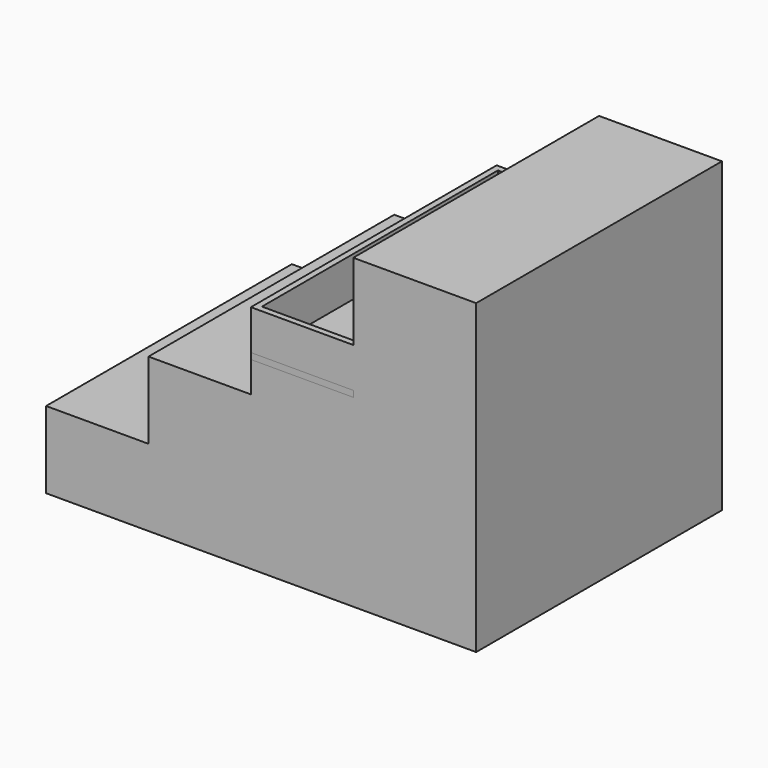
from build123d import *

# Parameters (mm, degrees)
F1_DEPTH = 60
F2_W     = 17.6
F2_H     = 57.6
F3_DEPTH = 25
F4_DEPTH = 16
F5_W     = 20
F5_H     = 60
F5_W_2   = 17.6
F5_H_2   = 57.6
F6_DEPTH = 1.2


with BuildPart() as f1:
    # F0 (on Front) → F1 (new body)
    with BuildSketch(Plane.XZ):
        Polygon((-84, 0), (0, 0), (0, 60), (-24, 60), (-24, 45), (-44, 45), (-44, 30), (-64, 30), (-64, 15), (-84, 15), align=None)
    extrude(amount=F1_DEPTH)

    # F2 (on face) → F3 (cut)
    with BuildSketch(Plane.XY.offset(45)):
        with Locations((-34, -30)):
            Rectangle(F2_W, F2_H)
    extrude(amount=-F3_DEPTH, mode=Mode.SUBTRACT)


with BuildPart() as f4:
    # F4 (new): a face of the model
    f4_faces = [f1.part.faces().sort_by_distance(p)[0] for p in [
        (-34, -30, 20),
    ]]
    extrude(f4_faces, amount=F4_DEPTH)

    # F5 (on face) → F6 (join)
    with BuildSketch(Plane.XY.offset(36)):
        with Locations((-34, -30)):
            Rectangle(F5_W, F5_H)
        with Locations((-34, -30)):
            Rectangle(F5_W_2, F5_H_2, mode=Mode.SUBTRACT)
        with Locations((-34, -30)):
            Rectangle(F5_W_2, F5_H_2)
    extrude(amount=F6_DEPTH)


solid = Compound([f1.part, f4.part])
